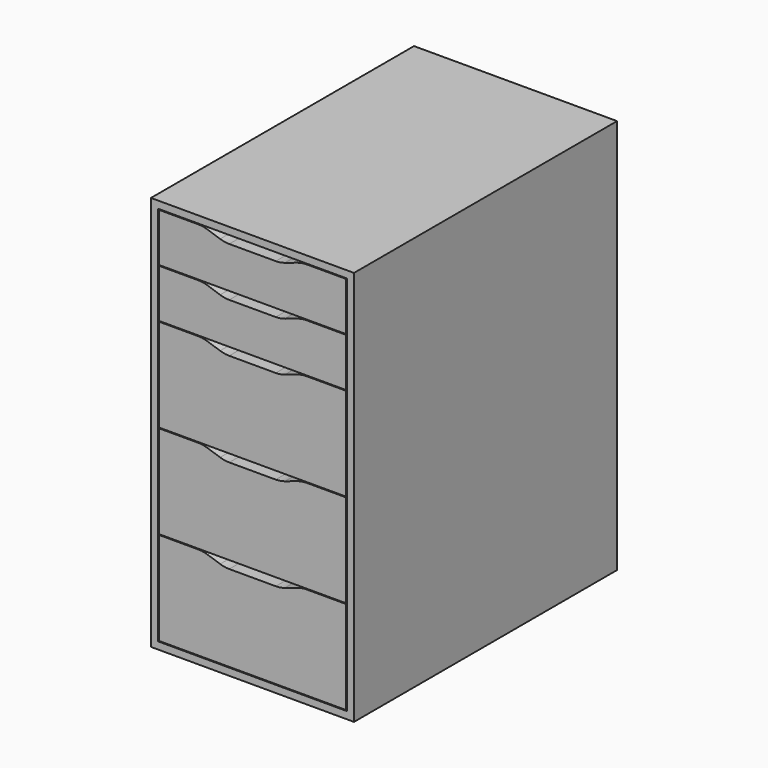
from build123d import *

# Parameters (mm, degrees)
F0_W      = 358.775
F0_H      = 698.5
F1_DEPTH  = 581.025
F2_W      = 333.375
F2_H      = 673.1
F2_W_2    = 330.835
F2_H_2    = 670.56
F3_DEPTH  = 304.8
F4_W      = 330.835
F4_H      = 1.27
F4_W_2    = 333.375
F4_W_3    = 332.105
F5_DEPTH  = 304.8
F7_DEPTH  = 304.8
F8_R      = 50.8
F10_DEPTH = 304.8
F11_R     = 50.8
F13_DEPTH = 304.8
F14_R     = 50.8
F16_DEPTH = 304.8
F17_R     = 50.8
F19_DEPTH = 304.8
F20_R     = 50.8


with BuildPart() as f1:
    # F0 (on Front) → F1 (new body)
    with BuildSketch(Plane.XZ):
        with Locations((130.6179589152, 307.5007573068)):
            Rectangle(F0_W, F0_H)
    extrude(amount=F1_DEPTH)

    # F2 (on face) → F3 (cut)
    with BuildSketch(Plane.XZ.offset(581.025)):
        with Locations((130.6179589152, 307.5007573068)):
            Rectangle(F2_W, F2_H)
        with Locations((130.6179589152, 307.5007573068)):
            Rectangle(F2_W_2, F2_H_2, mode=Mode.SUBTRACT)
    extrude(amount=-F3_DEPTH, mode=Mode.SUBTRACT)

    # F4 (on face) → F5 (cut)
    with BuildSketch(Plane.XZ.offset(581.025)):
        with Locations((130.6179589152, 556.4207573068)):
            Rectangle(F4_W, F4_H)
        with Locations((130.6179589152, 469.4257573068)):
            Rectangle(F4_W_2, F4_H)
        with Locations((129.9829589152, 303.5637573068)):
            Rectangle(F4_W_3, F4_H)
        with Locations((131.2529589152, 137.7017573068)):
            Rectangle(F4_W_3, F4_H)
    extrude(amount=-F5_DEPTH, mode=Mode.SUBTRACT)

    # F6 (on face) → F7 (cut)
    with BuildSketch(Plane.XZ.offset(581.025)):
        Polygon((218.0892089152, 642.7807573068), (43.1467089152, 642.7807573068), (81.2467089152, 630.0807573068), (179.9892089152, 630.0807573068), align=None)
    extrude(amount=-F7_DEPTH, mode=Mode.SUBTRACT)

    # F8
    f8_edges = [f1.edges().sort_by_distance(p)[0] for p in [
        (43.146709, -428.625, 642.780757),
        (81.246709, -428.625, 630.080757),
        (179.989209, -428.625, 630.080757),
        (218.089209, -428.625, 642.780757),
    ]]
    fillet(f8_edges, radius=F8_R)

    # F9 (on face) → F10 (cut)
    with BuildSketch(Plane.XZ.offset(581.025)):
        Polygon((218.0892089152, 555.7857573068), (43.1467089152, 555.7857573068), (81.2467089152, 543.0857573068), (179.9892089152, 543.0857573068), align=None)
    extrude(amount=-F10_DEPTH, mode=Mode.SUBTRACT)

    # F11
    f11_edges = [f1.edges().sort_by_distance(p)[0] for p in [
        (43.146709, -428.625, 555.785757),
        (81.246709, -428.625, 543.085757),
        (218.089209, -428.625, 555.785757),
        (179.989209, -428.625, 543.085757),
    ]]
    fillet(f11_edges, radius=F11_R)

    # F12 (on face) → F13 (cut)
    with BuildSketch(Plane.XZ.offset(581.025)):
        Polygon((218.0892089152, 468.7907573068), (43.1467089152, 468.7907573068), (81.2467089152, 456.0907573068), (179.9892089152, 456.0907573068), align=None)
    extrude(amount=-F13_DEPTH, mode=Mode.SUBTRACT)

    # F14
    f14_edges = [f1.edges().sort_by_distance(p)[0] for p in [
        (43.146709, -428.625, 468.790757),
        (81.246709, -428.625, 456.090757),
        (179.989209, -428.625, 456.090757),
        (218.089209, -428.625, 468.790757),
    ]]
    fillet(f14_edges, radius=F14_R)

    # F15 (on face) → F16 (cut)
    with BuildSketch(Plane.XZ.offset(581.025)):
        Polygon((218.0892089152, 302.9287573068), (43.1467089152, 302.9287573068), (81.2467089152, 290.2287573068), (179.9892089152, 290.2287573068), align=None)
    extrude(amount=-F16_DEPTH, mode=Mode.SUBTRACT)

    # F17
    f17_edges = [f1.edges().sort_by_distance(p)[0] for p in [
        (43.146709, -428.625, 302.928757),
        (81.246709, -428.625, 290.228757),
        (179.989209, -428.625, 290.228757),
        (218.089209, -428.625, 302.928757),
    ]]
    fillet(f17_edges, radius=F17_R)

    # F18 (on face) → F19 (cut)
    with BuildSketch(Plane.XZ.offset(581.025)):
        Polygon((218.0892089152, 137.0667573068), (43.1467089152, 137.0667573068), (81.2467089152, 124.3667573068), (179.9892089152, 124.3667573068), align=None)
    extrude(amount=-F19_DEPTH, mode=Mode.SUBTRACT)

    # F20
    f20_edges = [f1.edges().sort_by_distance(p)[0] for p in [
        (43.146709, -428.625, 137.066757),
        (81.246709, -428.625, 124.366757),
        (179.989209, -428.625, 124.366757),
        (218.089209, -428.625, 137.066757),
    ]]
    fillet(f20_edges, radius=F20_R)


solid = f1.part
